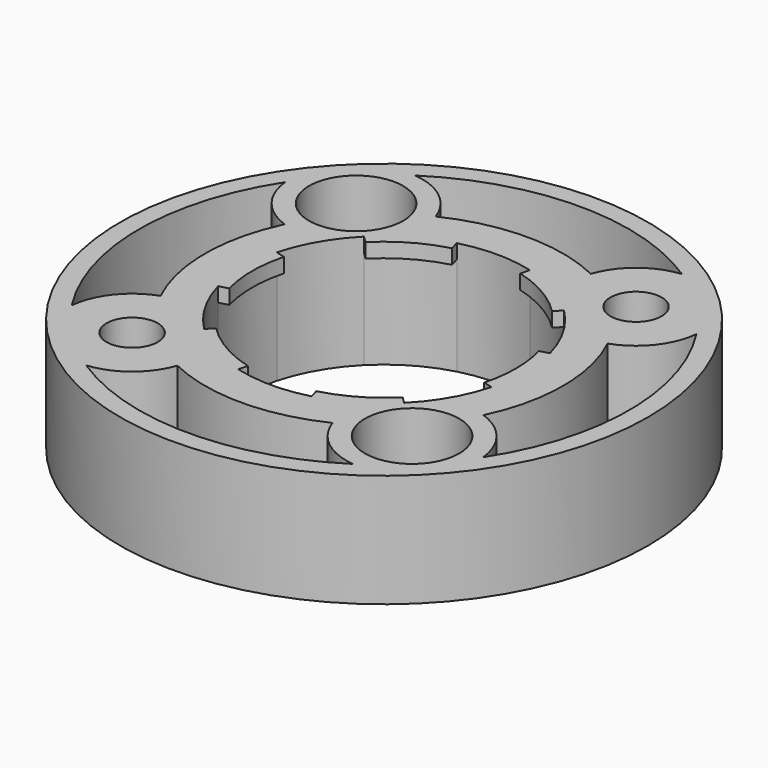
from build123d import *

# Parameters (mm, degrees)
F0_R             = 22.225
F0_R_2           = 2.15265
F1_DEPTH         = 9.525
F3_DEPTH         = 9.525
F4_COUNT         = 6
F4_ANGLE         = 300
F6_R             = 11.90625
F7_DEPTH         = 8.29945
F10_R            = 3.96875
F11_DEPTH        = 6.35
F12_R            = 3.96875
F13_DEPTH        = 6.35
F15_DEPTH        = 9.525
F15_COPIES_COUNT = 4


# Not quite as in the source:
# - a pattern or mirror of a feature is missing from the dataset's text; its kind, count and spacing are read off the source's solid


with BuildPart() as f1:
    # F0 (on Top) → F1 (new body)
    with BuildSketch(Plane.XY):
        Circle(F0_R)
        with Locations((-11.7865861589, -11.7865861589)):
            Circle(F0_R_2, mode=Mode.SUBTRACT)
        with Locations((11.7865861589, -11.7865861589)):
            Circle(F0_R_2, mode=Mode.SUBTRACT)
        with Locations((-11.7865861589, 11.7865861589)):
            Circle(F0_R_2, mode=Mode.SUBTRACT)
        with BuildLine():
            ThreePointArc((0, 11.1125), (7.8577241059, 7.8577241059), (11.1125, 0))
            ThreePointArc((11.1125, 0), (-7.8577241059, -7.8577241059), (0, 11.1125))
        make_face(mode=Mode.SUBTRACT)
        with Locations((11.7865861589, 11.7865861589)):
            Circle(F0_R_2, mode=Mode.SUBTRACT)
    extrude(amount=F1_DEPTH)

    # F2 (on face) → F3 (cut, through all)
    with BuildSketch(Plane.XY.offset(9.525)):
        with BuildLine():
            ThreePointArc((-2.8761266387, 10.7338507446), (0, 11.1125), (2.8761266387, 10.7338507446))
            Line((2.8761266387, 10.7338507446), (3.0815642558, 11.5005543693))
            ThreePointArc((3.0815642558, 11.5005543693), (0, 11.90625), (-3.0815642558, 11.5005543693))
            Line((-3.0815642558, 11.5005543693), (-2.8761266387, 10.7338507446))
        make_face()
    f3 = extrude(amount=-F3_DEPTH, mode=Mode.SUBTRACT)

    # F4: F3 ×6 about axis
    f4_axis = Axis((0, 0, 0), (0, 0, -1))
    for i in range(1, F4_COUNT):
        add(f3.rotate(f4_axis, i * F4_ANGLE / (F4_COUNT - 1)), mode=Mode.SUBTRACT)

    # F6 (on face) → F7 (cut, through all)
    with BuildSketch(Plane(origin=(0, 0, 0), x_dir=(1, 0, 0), z_dir=(0, 0, -1))):
        Circle(F6_R)
    extrude(amount=-F7_DEPTH, mode=Mode.SUBTRACT)

    # F10 (on face) → F11 (cut, through all)
    with BuildSketch(Plane(origin=(0, 0, 0), x_dir=(1, 0, 0), z_dir=(0, 0, -1))):
        with Locations((11.7865861589, -11.7865861589)):
            Circle(F10_R)
        with Locations((-11.7865861589, 11.7865861589)):
            Circle(F10_R)
    extrude(amount=-F11_DEPTH, mode=Mode.SUBTRACT)

    # F12 (on face) → F13 (cut, through all)
    with BuildSketch(Plane.XY.offset(9.525)):
        with Locations((-11.7865861589, 11.7865861589)):
            Circle(F12_R)
        with Locations((11.7865861589, -11.7865861589)):
            Circle(F12_R)
    extrude(amount=-F13_DEPTH, mode=Mode.SUBTRACT)

    # F14 (on face) → F15 (cut, through all)
    with BuildSketch(Plane(origin=(0, 0, 0), x_dir=(1, 0, 0), z_dir=(0, 0, -1))):
        with BuildLine():
            ThreePointArc((-11.229543123, 17.3148424047), (-8.3361072587, 16.1415958514), (-6.5322351826, 13.5931602316))
            ThreePointArc((-6.5322351826, 13.5931602316), (0, 15.08125), (6.5322351826, 13.5931602316))
            ThreePointArc((6.5322351826, 13.5931602316), (8.3361072587, 16.1415958514), (11.229543123, 17.3148424047))
            ThreePointArc((11.229543123, 17.3148424047), (0, 20.6375), (-11.229543123, 17.3148424047))
        make_face()
    f15 = extrude(amount=-F15_DEPTH, mode=Mode.SUBTRACT)

    # F15_copies: F15 ×4 about axis
    f15_copies_axis = Axis((0, 0, 0), (0, 0, 1))
    for i in range(1, F15_COPIES_COUNT):
        add(f15.rotate(f15_copies_axis, i * 360 / F15_COPIES_COUNT), mode=Mode.SUBTRACT)


solid = f1.part
